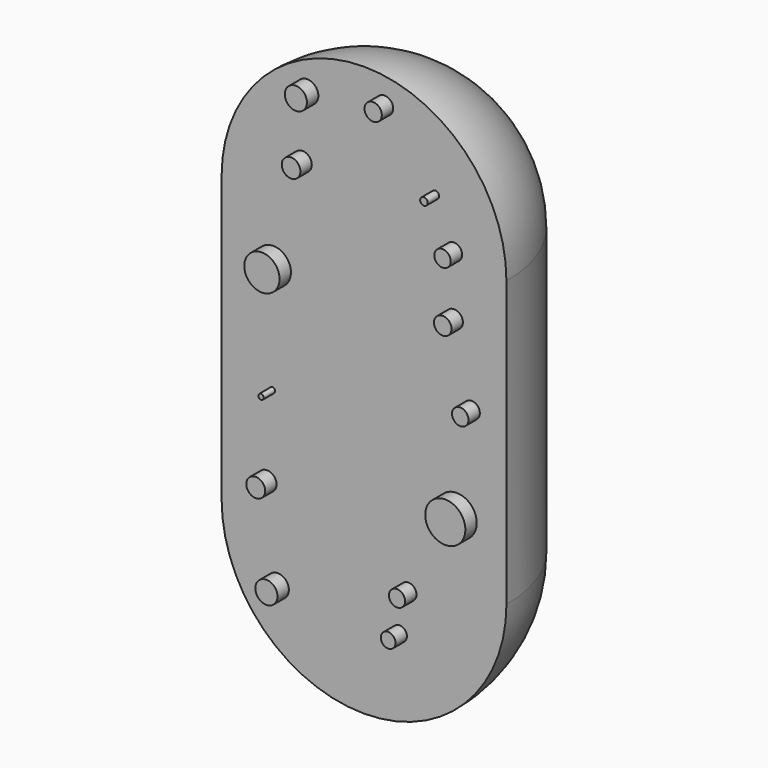
from build123d import *

# Parameters (mm, degrees)
F0_W     = 10
F0_H     = 20
F1_ANGLE = 180
F2_R     = 0.6542669189
F2_R_2   = 0.5762174249
F2_R_3   = 1.2390393019
F2_R_4   = 1.4098966941
F2_R_5   = 0.189897881
F2_R_6   = 0.6151811848
F2_R_7   = 0.7778029264
F2_R_8   = 0.6623255224
F2_R_9   = 0.6070903234
F2_R_10  = 0.7783808961
F2_R_11  = 0.265053414
F2_R_12  = 0.5177294077
F2_R_13  = 0.5684145952
F2_R_14  = 0.5786464401
F4_DEPTH = 1


# Not quite as in the source:
# - the program builds the solid bodies; features that only make, move or delete a surface that nothing else refers to are left out


with BuildPart() as f1:
    # F0 (on Front) → F1 (revolve)
    with BuildSketch(Plane.XZ):
        with Locations((5, 10)):
            Rectangle(F0_W, F0_H)
        with BuildLine():
            Line((10, 0), (0, 0))
            ThreePointArc((0, 0), (2.9289321881, -7.0710678119), (10, -10))
            Line((10, -10), (10, 0))
        make_face()
        with BuildLine():
            ThreePointArc((10, 30), (2.9289321881, 27.0710678119), (0, 20))
            Line((0, 20), (10, 20))
            Line((10, 20), (10, 30))
        make_face()
    revolve(axis=Axis((10, 0, 10), (0, 0, -1)), revolution_arc=F1_ANGLE)

    # F2 (on face) → F4 (join)
    with BuildSketch(Plane.XZ):
        with Locations((5.6774760596, 22.7308552712)):
            Circle(F2_R)
        with Locations((16.3127072155, 20.606238395)):
            Circle(F2_R_2)
        with Locations((3.6300569773, 15.6070627272)):
            Circle(F2_R_3)
        with Locations((16.507089138, 4.3547041714)):
            Circle(F2_R_4)
        with Locations((3.5698860884, 7.9049132764)):
            Circle(F2_R_5)
        with Locations((16.3283385336, 16.4442379028)):
            Circle(F2_R_6)
        with Locations((3.9457399398, -4.0635056794)):
            Circle(F2_R_7)
        with Locations((3.19618918, 2.172768116)):
            Circle(F2_R_8)
        with Locations((11.4412605762, 28.0772857368)):
            Circle(F2_R_9)
        with Locations((6.0145035386, 27.1478407085)):
            Circle(F2_R_10)
        with Locations((15.0091275573, 23.699901998)):
            Circle(F2_R_11)
        with Locations((12.4958753586, -4.2460225523)):
            Circle(F2_R_12)
        with Locations((13.1159704179, -1.4507770538)):
            Circle(F2_R_13)
        with Locations((17.5564400852, 11.2137598917)):
            Circle(F2_R_14)
    extrude(amount=F4_DEPTH)


solid = f1.part
